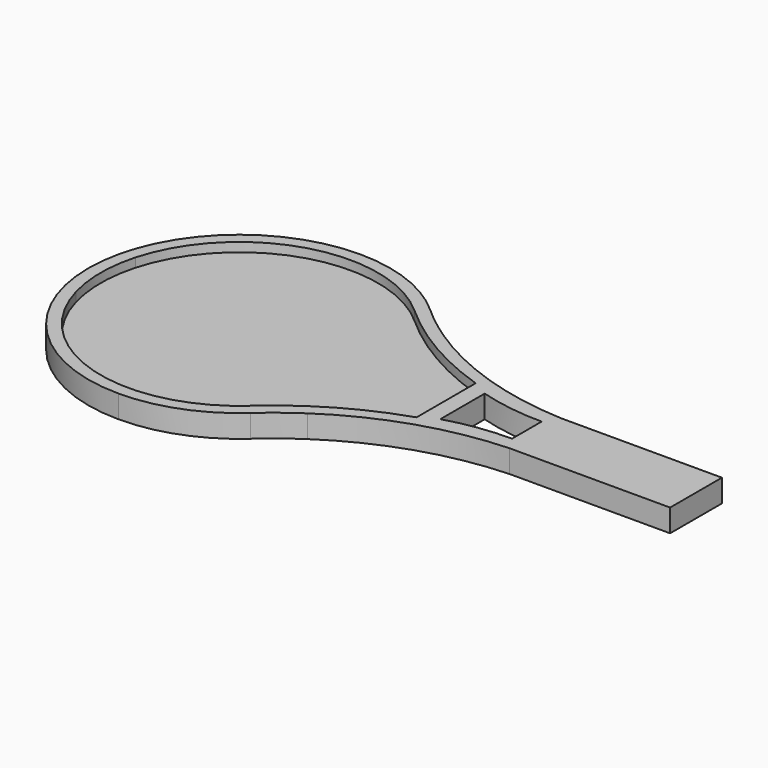
from build123d import *

# Parameters (mm, degrees)
F0_W     = 29.9560762942
F0_H     = 7.1370224468
F0_W_2   = 35.3452544659
F1_DEPTH = 5
F2_W     = 3.7603338286
F2_H     = 4.0725159595
F2_W_2   = 14.1769461334
F3_DEPTH = 2
F4_DEPTH = 25


with BuildPart() as f1:
    # F0 (on Top) → F1 (new body)
    with BuildSketch(Plane.XY):
        with BuildLine():
            Line((0, 7.1370224468), (0, 33.2578741251))
            ThreePointArc((0, 33.2578741251), (-23.5168683217, 23.5168683217), (-33.2578741251, 0))
            Line((-33.2578741251, 0), (-29.9560762942, 0))
            Line((-29.9560762942, 0), (-29.9560762942, 7.1370224468))
            Line((-29.9560762942, 7.1370224468), (0, 7.1370224468))
        make_face()
        with BuildLine():
            Line((-29.9560762942, 0), (-33.2578741251, 0))
            ThreePointArc((-33.2578741251, 0), (-23.5168683217, -23.5168683217), (0, -33.2578741251))
            Line((0, -33.2578741251), (0, -7.1370224468))
            Line((0, -7.1370224468), (-29.9560762942, -7.1370224468))
            Line((-29.9560762942, -7.1370224468), (-29.9560762942, 0))
        make_face()
        with Locations((-14.9780381471, -3.5685112234)):
            Rectangle(F0_W, F0_H)
        with Locations((-14.9780381471, 3.5685112234)):
            Rectangle(F0_W, F0_H)
        with BuildLine():
            Line((0, -7.1370224468), (0, -33.2578741251))
            ThreePointArc((0, -33.2578741251), (11.9212758791, -31.0478561697), (22.2581910956, -24.7115179719))
            Line((22.2581910956, -24.7115179719), (6.4284682817, -7.1370224468))
            Line((6.4284682817, -7.1370224468), (0, -7.1370224468))
        make_face()
        with BuildLine():
            Line((29.9560762942, -7.1370224468), (6.4284682817, -7.1370224468))
            Line((6.4284682817, -7.1370224468), (22.2581910956, -24.7115179719))
            ThreePointArc((22.2581910956, -24.7115179719), (26.6068003283, -19.95405642), (29.9560762942, -14.4471341234))
            Line((29.9560762942, -14.4471341234), (29.9560762942, -7.1370224468))
        make_face()
        Polygon((6.4284682817, -7.1370224468), (0, 0), (0, -7.1370224468), align=None)
        Polygon((29.9560762942, 0), (0, 0), (6.4284682817, -7.1370224468), (29.9560762942, -7.1370224468), align=None)
        Polygon((29.9560762942, 7.1370224468), (6.4284682817, 7.1370224468), (0, 0), (29.9560762942, 0), align=None)
        Polygon((0, 0), (6.4284682817, 7.1370224468), (0, 7.1370224468), align=None)
        with BuildLine():
            ThreePointArc((29.9560762942, 14.4471341234), (26.6068003283, 19.95405642), (22.2581910956, 24.7115179719))
            Line((22.2581910956, 24.7115179719), (6.4284682817, 7.1370224468))
            Line((6.4284682817, 7.1370224468), (29.9560762942, 7.1370224468))
            Line((29.9560762942, 7.1370224468), (29.9560762942, 14.4471341234))
        make_face()
        with BuildLine():
            Line((6.4284682817, 7.1370224468), (22.2581910956, 24.7115179719))
            ThreePointArc((22.2581910956, 24.7115179719), (11.9212758791, 31.0478561697), (0, 33.2578741251))
            Line((0, 33.2578741251), (0, 7.1370224468))
            Line((0, 7.1370224468), (6.4284682817, 7.1370224468))
        make_face()
        with BuildLine():
            ThreePointArc((29.9560762942, 18.7118758373), (26.0003436233, 21.5746791136), (22.2581910956, 24.7115179719))
            ThreePointArc((22.2581910956, 24.7115179719), (26.6068003283, 19.95405642), (29.9560762942, 14.4471341234))
            Line((29.9560762942, 14.4471341234), (29.9560762942, 18.7118758373))
        make_face()
        with BuildLine():
            ThreePointArc((29.9560762942, -14.4471341234), (26.6068003283, -19.95405642), (22.2581910956, -24.7115179719))
            ThreePointArc((22.2581910956, -24.7115179719), (26.0003436233, -21.5746791136), (29.9560762942, -18.7118758373))
            Line((29.9560762942, -18.7118758373), (29.9560762942, -14.4471341234))
        make_face()
        with BuildLine():
            ThreePointArc((29.9560762942, -14.4471341234), (31.4327985964, -10.8657886838), (32.4830586909, -7.1370224468))
            Line((32.4830586909, -7.1370224468), (29.9560762942, -7.1370224468))
            Line((29.9560762942, -7.1370224468), (29.9560762942, -14.4471341234))
        make_face()
        with BuildLine():
            ThreePointArc((32.4830586909, -7.1370224468), (33.0636028622, -3.5894786656), (33.2578741251, 0))
            Line((33.2578741251, 0), (29.9560762942, 0))
            Line((29.9560762942, 0), (29.9560762942, -7.1370224468))
            Line((29.9560762942, -7.1370224468), (32.4830586909, -7.1370224468))
        make_face()
        with BuildLine():
            ThreePointArc((33.2578741251, 0), (33.0636028622, 3.5894786656), (32.4830586909, 7.1370224468))
            Line((32.4830586909, 7.1370224468), (29.9560762942, 7.1370224468))
            Line((29.9560762942, 7.1370224468), (29.9560762942, 0))
            Line((29.9560762942, 0), (33.2578741251, 0))
        make_face()
        with BuildLine():
            ThreePointArc((32.4830586909, 7.1370224468), (31.4327985964, 10.8657886838), (29.9560762942, 14.4471341234))
            Line((29.9560762942, 14.4471341234), (29.9560762942, 7.1370224468))
            Line((29.9560762942, 7.1370224468), (32.4830586909, 7.1370224468))
        make_face()
        with BuildLine():
            Line((29.9560762942, 18.7118758373), (29.9560762942, 14.4471341234))
            ThreePointArc((29.9560762942, 14.4471341234), (31.4327985964, 10.8657886838), (32.4830586909, 7.1370224468))
            Line((32.4830586909, 7.1370224468), (65.3013307601, 7.1370224468))
            ThreePointArc((65.3013307601, 7.1370224468), (46.829633004, 10.4843879142), (29.9560762942, 18.7118758373))
        make_face()
        with BuildLine():
            Line((65.3013307601, 7.1370224468), (32.4830586909, 7.1370224468))
            ThreePointArc((32.4830586909, 7.1370224468), (33.0636028622, 3.5894786656), (33.2578741251, 0))
            Line((33.2578741251, 0), (65.3013307601, 0))
            Line((65.3013307601, 0), (65.3013307601, 7.1370224468))
        make_face()
        with BuildLine():
            Line((65.3013307601, 0), (33.2578741251, 0))
            ThreePointArc((33.2578741251, 0), (33.0636028622, -3.5894786656), (32.4830586909, -7.1370224468))
            Line((32.4830586909, -7.1370224468), (65.3013307601, -7.1370224468))
            Line((65.3013307601, -7.1370224468), (65.3013307601, 0))
        make_face()
        with BuildLine():
            Line((65.3013307601, -7.1370224468), (32.4830586909, -7.1370224468))
            ThreePointArc((32.4830586909, -7.1370224468), (31.4327985964, -10.8657886838), (29.9560762942, -14.4471341234))
            Line((29.9560762942, -14.4471341234), (29.9560762942, -18.7118758373))
            ThreePointArc((29.9560762942, -18.7118758373), (46.829633004, -10.4843879142), (65.3013307601, -7.1370224468))
        make_face()
        with Locations((82.9739579931, -3.5685112234)):
            Rectangle(F0_W_2, F0_H)
        with Locations((82.9739579931, 3.5685112234)):
            Rectangle(F0_W_2, F0_H)
    extrude(amount=F1_DEPTH)

    # F2 (on face) → F3 (cut)
    with BuildSketch(Plane.XY.offset(5)):
        with BuildLine():
            Line((7.3364039044, 8.145031919), (29.4496861323, 8.145031919))
            ThreePointArc((29.4496861323, 8.145031919), (25.9897625324, 16.0672898076), (20.4494554433, 22.703421115))
            Line((20.4494554433, 22.703421115), (7.3364039044, 8.145031919))
        make_face()
        with BuildLine():
            Line((45.5672070233, 8.145031919), (29.4496861323, 8.145031919))
            ThreePointArc((29.4496861323, 8.145031919), (29.9355135784, 6.1229555814), (30.2826711505, 4.0725159595))
            Line((30.2826711505, 4.0725159595), (45.5672070233, 4.0725159595))
            Line((45.5672070233, 4.0725159595), (45.5672070233, 5.9387854649))
            Line((45.5672070233, 5.9387854649), (45.5672070233, 8.145031919))
        make_face()
        Polygon((29.4496861323, 4.0725159595), (29.4496861323, 8.145031919), (7.3364039044, 8.145031919), (3.6682019522, 4.0725159595), (25.6893523037, 4.0725159595), align=None)
        with BuildLine():
            ThreePointArc((30.2826711505, 4.0725159595), (29.9355135784, 6.1229555814), (29.4496861323, 8.145031919))
            Line((29.4496861323, 8.145031919), (29.4496861323, 4.0725159595))
            Line((29.4496861323, 4.0725159595), (30.2826711505, 4.0725159595))
        make_face()
        with BuildLine():
            ThreePointArc((20.4494554433, 22.703421115), (25.9897625324, 16.0672898076), (29.4496861323, 8.145031919))
            Line((29.4496861323, 8.145031919), (45.5672070233, 8.145031919))
            ThreePointArc((45.5672070233, 8.145031919), (32.2488302064, 14.1138509074), (20.4494554433, 22.703421115))
        make_face()
        with BuildLine():
            Line((7.3364039044, 8.145031919), (20.4494554433, 22.703421115))
            ThreePointArc((20.4494554433, 22.703421115), (-8.557903488, 29.3323685737), (-29.4496861323, 8.145031919))
            Line((-29.4496861323, 8.145031919), (7.3364039044, 8.145031919))
        make_face()
        with BuildLine():
            Line((45.5672070233, 4.0725159595), (30.2826711505, 4.0725159595))
            ThreePointArc((30.2826711505, 4.0725159595), (30.4870567923, 2.0408151309), (30.5552869116, 0))
            Line((30.5552869116, 0), (45.5672070233, 0))
            Line((45.5672070233, 0), (45.5672070233, 4.0725159595))
        make_face()
        with BuildLine():
            ThreePointArc((30.5552869116, 0), (30.4870567923, 2.0408151309), (30.2826711505, 4.0725159595))
            Line((30.2826711505, 4.0725159595), (29.4496861323, 4.0725159595))
            Line((29.4496861323, 4.0725159595), (29.4496861323, 0))
            Line((29.4496861323, 0), (30.5552869116, 0))
        make_face()
        Polygon((3.6682019522, 4.0725159595), (7.3364039044, 8.145031919), (-29.4496861323, 8.145031919), (-29.4496861323, -8.145031919), (7.3364039044, -8.145031919), (3.6682019522, -4.0725159595), (-25.6893523037, -4.0725159595), (-25.6893523037, 4.0725159595), align=None)
        with Locations((27.569519218, 2.0362579798)):
            Rectangle(F2_W, F2_H)
        with BuildLine():
            Line((-29.4496861323, -8.145031919), (-29.4496861323, 8.145031919))
            ThreePointArc((-29.4496861323, 8.145031919), (-30.5552869116, 0), (-29.4496861323, -8.145031919))
        make_face()
        with BuildLine():
            Line((45.5672070233, 0), (30.5552869116, 0))
            ThreePointArc((30.5552869116, 0), (30.4870567923, -2.0408151309), (30.2826711505, -4.0725159595))
            Line((30.2826711505, -4.0725159595), (45.5672070233, -4.0725159595))
            Line((45.5672070233, -4.0725159595), (45.5672070233, 0))
        make_face()
        with BuildLine():
            ThreePointArc((30.2826711505, -4.0725159595), (30.4870567923, -2.0408151309), (30.5552869116, 0))
            Line((30.5552869116, 0), (29.4496861323, 0))
            Line((29.4496861323, 0), (29.4496861323, -4.0725159595))
            Line((29.4496861323, -4.0725159595), (30.2826711505, -4.0725159595))
        make_face()
        Polygon((25.6893523037, 4.0725159595), (3.6682019522, 4.0725159595), (0, 0), (25.6893523037, 0), align=None)
        Polygon((0, 0), (3.6682019522, 4.0725159595), (-25.6893523037, 4.0725159595), (-25.6893523037, -4.0725159595), (3.6682019522, -4.0725159595), align=None)
        with Locations((27.569519218, -2.0362579798)):
            Rectangle(F2_W, F2_H)
        with BuildLine():
            Line((7.3364039044, -8.145031919), (-29.4496861323, -8.145031919))
            ThreePointArc((-29.4496861323, -8.145031919), (-8.557903488, -29.3323685737), (20.4494554433, -22.703421115))
            Line((20.4494554433, -22.703421115), (7.3364039044, -8.145031919))
        make_face()
        with BuildLine():
            Line((45.5672070233, -4.0725159595), (30.2826711505, -4.0725159595))
            ThreePointArc((30.2826711505, -4.0725159595), (29.9355135784, -6.1229555814), (29.4496861323, -8.145031919))
            Line((29.4496861323, -8.145031919), (45.5672070233, -8.145031919))
            Line((45.5672070233, -8.145031919), (45.5672070233, -5.9387854649))
            Line((45.5672070233, -5.9387854649), (45.5672070233, -4.0725159595))
        make_face()
        with BuildLine():
            ThreePointArc((29.4496861323, -8.145031919), (29.9355135784, -6.1229555814), (30.2826711505, -4.0725159595))
            Line((30.2826711505, -4.0725159595), (29.4496861323, -4.0725159595))
            Line((29.4496861323, -4.0725159595), (29.4496861323, -8.145031919))
        make_face()
        with BuildLine():
            Line((49.188118428, 6.1087739393), (49.188118428, 4.0725159595))
            Line((49.188118428, 4.0725159595), (63.3650645614, 4.0725159595))
            ThreePointArc((63.3650645614, 4.0725159595), (56.2038469933, 4.5841792227), (49.188118428, 6.1087739393))
        make_face()
        with Locations((56.2765914947, 2.0362579798)):
            Rectangle(F2_W_2, F2_H)
        Polygon((25.6893523037, 0), (0, 0), (3.6682019522, -4.0725159595), (25.6893523037, -4.0725159595), align=None)
        Polygon((29.4496861323, -8.145031919), (29.4496861323, -4.0725159595), (25.6893523037, -4.0725159595), (3.6682019522, -4.0725159595), (7.3364039044, -8.145031919), align=None)
        with BuildLine():
            Line((7.3364039044, -8.145031919), (20.4494554433, -22.703421115))
            ThreePointArc((20.4494554433, -22.703421115), (25.9897625324, -16.0672898076), (29.4496861323, -8.145031919))
            Line((29.4496861323, -8.145031919), (7.3364039044, -8.145031919))
        make_face()
        with BuildLine():
            ThreePointArc((29.4496861323, -8.145031919), (25.9897625324, -16.0672898076), (20.4494554433, -22.703421115))
            ThreePointArc((20.4494554433, -22.703421115), (32.2488302064, -14.1138509074), (45.5672070233, -8.145031919))
            Line((45.5672070233, -8.145031919), (29.4496861323, -8.145031919))
        make_face()
        with Locations((56.2765914947, -2.0362579798)):
            Rectangle(F2_W_2, F2_H)
        with BuildLine():
            Line((63.3650645614, -4.0725159595), (49.188118428, -4.0725159595))
            Line((49.188118428, -4.0725159595), (49.188118428, -6.1087739393))
            ThreePointArc((49.188118428, -6.1087739393), (56.2038469933, -4.5841792227), (63.3650645614, -4.0725159595))
        make_face()
    extrude(amount=-F3_DEPTH, mode=Mode.SUBTRACT)

    # F4 (cut): a face of the model
    f4_faces = [f1.faces().sort_by_distance(p)[0] for p in [
        (55.7717921827, 0, 3),
    ]]
    extrude(f4_faces, amount=-F4_DEPTH, mode=Mode.SUBTRACT)


solid = f1.part
